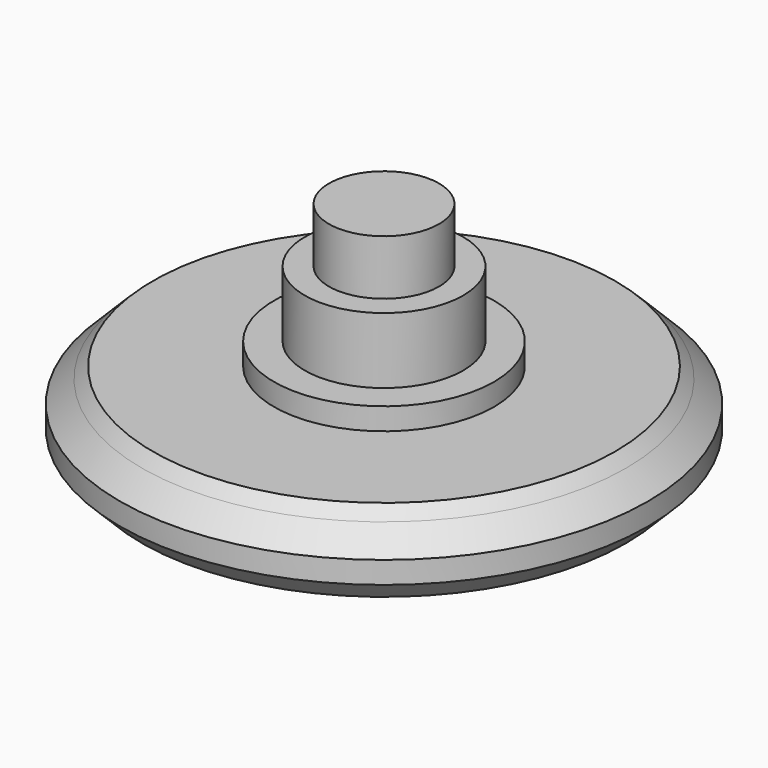
from build123d import *

# Parameters (mm, degrees)
F0_R      = 12
F0_R_2    = 11
F0_R_3    = 5
F0_R_4    = 4.1
F0_R_5    = 3
F1_DEPTH  = 2
F2_DEPTH  = 3.5
F3_SIZE   = 0.99999
F4_DEPTH  = 4.5
F5_DEPTH  = 7.5
F6_DEPTH  = 10
F7_SIZE   = 1
F8_SIZE   = 0.5
F9_R      = 3
F9_R_2    = 2.5
F10_DEPTH = 2.5
F11_R     = 4.1
F11_R_2   = 3.6
F12_DEPTH = 3


# Not quite as in the source:
# - a fillet or chamfer is up to 0.001 mm smaller than in the source, because OpenCascade refuses the exact size


with BuildPart() as f1:
    # F0 (on Top) → F1 (new body)
    with BuildSketch(Plane.XY):
        Circle(F0_R)
        Circle(F0_R_2, mode=Mode.SUBTRACT)
        Circle(F0_R_2)
        Circle(F0_R_3, mode=Mode.SUBTRACT)
        Circle(F0_R_3)
        Circle(F0_R_4, mode=Mode.SUBTRACT)
        Circle(F0_R_4)
        Circle(F0_R_5, mode=Mode.SUBTRACT)
        Circle(F0_R_5)
    extrude(amount=F1_DEPTH)

    # F0 (on Top) → F2 (join)
    with BuildSketch(Plane.XY):
        Circle(F0_R_2)
        Circle(F0_R_3, mode=Mode.SUBTRACT)
        Circle(F0_R_3)
        Circle(F0_R_4, mode=Mode.SUBTRACT)
        Circle(F0_R_4)
        Circle(F0_R_5, mode=Mode.SUBTRACT)
        Circle(F0_R_5)
    extrude(amount=F2_DEPTH)

    # F3 (size 1 in the source; OpenCascade refuses exactly that, so slightly less here)
    f3_edges = [f1.edges().sort_by_distance(p)[0] for p in [
        (-11, 0, 2),
    ]]
    chamfer(f3_edges, length=F3_SIZE)

    # F0 (on Top) → F4 (join)
    with BuildSketch(Plane.XY):
        Circle(F0_R_3)
        Circle(F0_R_4, mode=Mode.SUBTRACT)
        Circle(F0_R_4)
        Circle(F0_R_5, mode=Mode.SUBTRACT)
        Circle(F0_R_5)
    extrude(amount=F4_DEPTH)

    # F0 (on Top) → F5 (join)
    with BuildSketch(Plane.XY):
        Circle(F0_R_4)
        Circle(F0_R_5, mode=Mode.SUBTRACT)
    extrude(amount=F5_DEPTH)

    # F0 (on Top) → F6 (join)
    with BuildSketch(Plane.XY):
        Circle(F0_R_5)
    extrude(amount=F6_DEPTH)

    # F7
    f7_edges = [f1.edges().sort_by_distance(p)[0] for p in [
        (-12, 0, 0),
    ]]
    chamfer(f7_edges, length=F7_SIZE)

    # F8
    f8_edges = [f1.edges().sort_by_distance(p)[0] for p in [
        (-11, 0, 3.5),
    ]]
    chamfer(f8_edges, length=F8_SIZE)

    # F9 (on face) → F10 (cut, through all)
    with BuildSketch(Plane.XY.offset(10)):
        Circle(F9_R)
        Circle(F9_R_2, mode=Mode.SUBTRACT)
    extrude(amount=-F10_DEPTH, mode=Mode.SUBTRACT)

    # F11 (on face) → F12 (cut, through all)
    with BuildSketch(Plane.XY.offset(7.5)):
        Circle(F11_R)
        Circle(F11_R_2, mode=Mode.SUBTRACT)
    extrude(amount=-F12_DEPTH, mode=Mode.SUBTRACT)


solid = f1.part
